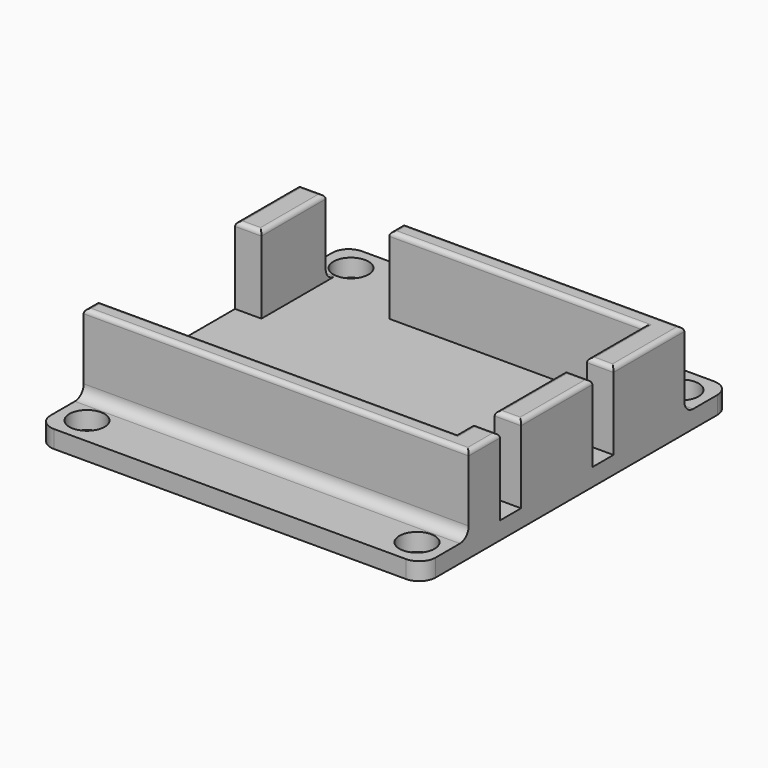
from build123d import *

# Parameters (mm, degrees)
F0_R     = 1.6
F1_DEPTH = 1.6
F2_W     = 2.4
F2_H     = 8.1
F2_H_2   = 1.65
F3_DEPTH = 7
F4_R     = 1
F5_R     = 0.4


with BuildPart() as f1:
    # F0 (on Top) → F1 (new body)
    with BuildSketch(Plane.XY):
        with BuildLine():
            ThreePointArc((-17.5, -16), (-17.0606601718, -17.0606601718), (-16, -17.5))
            Line((-16, -17.5), (16, -17.5))
            ThreePointArc((16, -17.5), (17.0606601718, -17.0606601718), (17.5, -16))
            Line((17.5, -16), (17.5, 16))
            ThreePointArc((17.5, 16), (17.0606601718, 17.0606601718), (16, 17.5))
            Line((16, 17.5), (-16, 17.5))
            ThreePointArc((-16, 17.5), (-17.0606601718, 17.0606601718), (-17.5, 16))
            Line((-17.5, 16), (-17.5, -16))
        make_face()
        with Locations((-15, -15)):
            Circle(F0_R, mode=Mode.SUBTRACT)
        with Locations((15, -15)):
            Circle(F0_R, mode=Mode.SUBTRACT)
        with Locations((-15, 15)):
            Circle(F0_R, mode=Mode.SUBTRACT)
        with Locations((15, 15)):
            Circle(F0_R, mode=Mode.SUBTRACT)
    extrude(amount=F1_DEPTH)

    # F2 (on face) → F3 (join)
    with BuildSketch(Plane.XY.offset(1.6)):
        Polygon((15.1, -10.6), (-15.1, -10.6), (-15.1, -12.25), (17.5, -12.25), (17.5, -8.7), (15.1, -8.7), align=None)
        with Locations((16.3, -2.25)):
            Rectangle(F2_W, F2_H)
        Polygon((-8, 12.25), (-8, 10.6), (15.1, 10.6), (15.1, 4.2), (17.5, 4.2), (17.5, 12.25), align=None)
        Polygon((-17.5, 4.95), (-15.1, 4.95), (-15.1, 10.6), (-15.1, 12.25), (-17.5, 12.25), align=None)
        with Locations((-16.3, -11.425)):
            Rectangle(F2_W, F2_H_2)
    extrude(amount=F3_DEPTH)

    # F4
    f4_edges = [f1.edges().sort_by_distance(p)[0] for p in [
        (0, -12.25, 1.6),
        (4.75, 12.25, 1.6),
        (-16.3, 12.25, 1.6),
    ]]
    fillet(f4_edges, radius=F4_R)

    # F5
    f5_edges = [f1.edges().sort_by_distance(p)[0] for p in [
        (4.75, 12.25, 8.6),
        (3.55, 10.6, 8.6),
        (-15.1, 8.6, 8.6),
        (-17.5, 8.6, 8.6),
        (-16.3, 12.25, 8.6),
        (-8, 11.425, 8.6),
        (-16.3, 4.95, 8.6),
        (-1.2, -10.6, 8.6),
        (0, -12.25, 8.6),
        (16.3, -8.7, 8.6),
        (17.5, -10.475, 8.6),
        (15.1, -9.65, 8.6),
        (16.3, -6.3, 8.6),
        (15.1, -2.25, 8.6),
        (17.5, -2.25, 8.6),
        (16.3, 1.8, 8.6),
        (16.3, 4.2, 8.6),
        (15.1, 7.4, 8.6),
        (17.5, 8.225, 8.6),
        (-17.5, -11.425, 8.6),
    ]]
    fillet(f5_edges, radius=F5_R)


solid = f1.part
